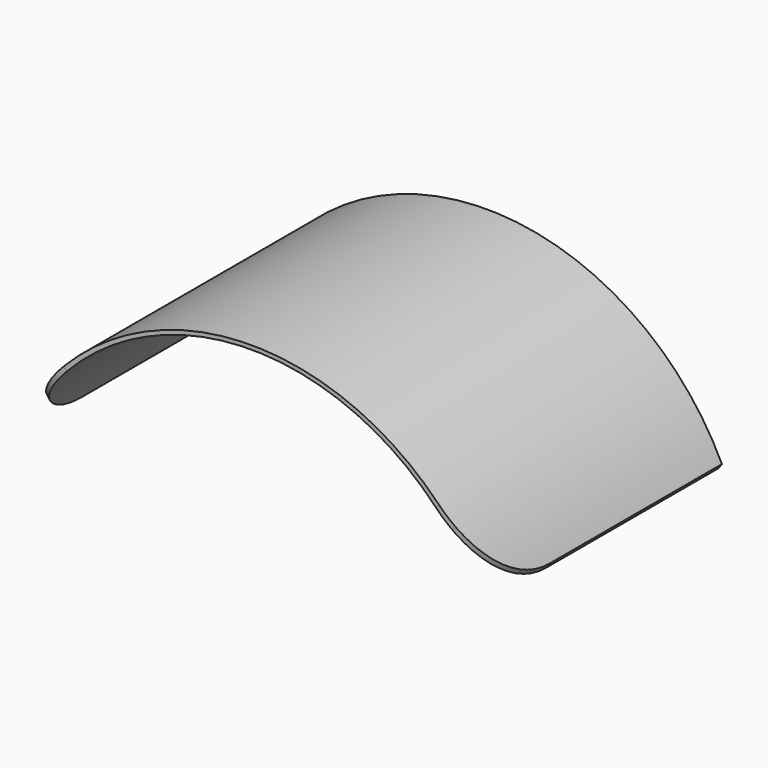
from build123d import *

# Parameters (mm, degrees)
F1_DEPTH    = 127
F2_T1_DEPTH = 340.4898987322
F2_T3_DEPTH = 340.4898987322


# Not quite as in the source:
# - a fillet or chamfer that OpenCascade refuses, or shapes differently, is made with other operations: its cross-section is extruded or revolved along the edge and cut away or added


with BuildPart() as f1:
    # F0 (on Front) → F1 (new body)
    with BuildSketch(Plane.XZ):
        with BuildLine():
            ThreePointArc((0, 0), (100, 64.1742430504), (200, 0))
            Line((200, 0), (201.4339410909, 2.0478801107))
            ThreePointArc((201.4339410909, 2.0478801107), (100, 65.8918877277), (-1.4339410909, 2.0478801107))
            Line((-1.4339410909, 2.0478801107), (0, 0))
        make_face()
    extrude(amount=F1_DEPTH)

    # F2: fillet of radius 33.7989898732 on 2 edges, made by hand

    # F2_s2 → F2_t1 (cut)
    with BuildSketch(Plane(origin=(-79.5992955607, 0, -113.6795752931), x_dir=(0, 1, 0), z_dir=(0.5735764364, 0, 0.8191520443))):
        with BuildLine():
            ThreePointArc((-93.2010101268, -163.8304088578), (-117.1005050634, -153.9309139212), (-127, -130.0314189846))
            Line((-127, -130.0314189846), (-127, -163.8304088578))
            Line((-127, -163.8304088578), (-93.2010101268, -163.8304088578))
        make_face()
    extrude(amount=F2_T1_DEPTH, mode=Mode.SUBTRACT)

    # F2_s4 → F2_t3 (cut)
    with BuildSketch(Plane(origin=(-49.8997015002, 0, 71.2641592346), x_dir=(0, 1, 0), z_dir=(0.5735764364, 0, -0.8191520443))):
        with BuildLine():
            ThreePointArc((-93.2010101268, 0), (-117.1005050634, 9.8994949366), (-127, 33.7989898732))
            Line((-127, 33.7989898732), (-127, 0))
            Line((-127, 0), (-93.2010101268, 0))
        make_face()
    extrude(amount=F2_T3_DEPTH, mode=Mode.SUBTRACT)


solid = f1.part
